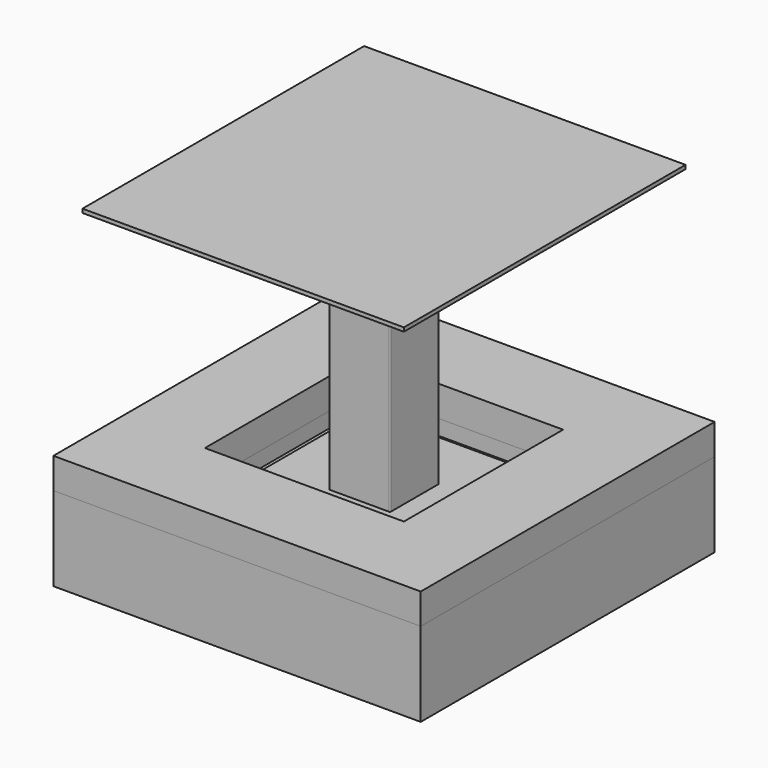
from build123d import *

# Parameters (mm, degrees)
F0_W           = 1219.2
F0_H           = 1219.2
F1_DEPTH       = 304.8
F2_DEPTH       = 25.4
F3_W           = 660.4
F3_H           = 660.4
F4_DEPTH       = 152.4
F5_W           = 660.4
F5_H           = 660.4
F6_DEPTH       = 101.6
F7_W           = 1219.2
F7_H           = 1219.2
F7_W_2         = 660.4
F7_H_2         = 660.4
F8_DEPTH       = 101.6
F9_W           = 609.6
F9_H           = 609.6
F10_DEPTH      = 12.7
F12_DEPTH      = 863.6
F13_W          = 1066.8
F13_H          = 1168.4
F14_DEPTH      = 12.7
F15_R          = 6.35
F16_DEPTH      = 76.2
F17_R          = 6.35
F18_DEPTH      = 50.8
F18_DEPTH_BACK = 12.7


with BuildPart() as f1:
    # F0 (on Top) → F1 (new body)
    with BuildSketch(Plane.XY):
        Rectangle(F0_W, F0_H)
    extrude(amount=-F1_DEPTH)

    # F2 (cut): a face of the model
    f2_faces = [f1.faces().sort_by_distance(p)[0] for p in [
        (0, 0, 0),
    ]]
    extrude(f2_faces, amount=-F2_DEPTH, mode=Mode.SUBTRACT)

    # F3 (on face) → F4 (cut)
    with BuildSketch(Plane.XY.offset(-25.4)):
        Rectangle(F3_W, F3_H)
    extrude(amount=-F4_DEPTH, mode=Mode.SUBTRACT)


with BuildPart() as f6:
    # F5 (on face) → F6 (new body)
    with BuildSketch(Plane.XY.offset(-177.8)):
        Rectangle(F5_W, F5_H)
    extrude(amount=F6_DEPTH)


with BuildPart() as f8:
    # F7 (on face) → F8 (new body)
    with BuildSketch(Plane.XY.offset(-25.4)):
        Rectangle(F7_W, F7_H)
        Rectangle(F7_W_2, F7_H_2, mode=Mode.SUBTRACT)
    extrude(amount=F8_DEPTH)


with BuildPart() as f10:
    # F9 (on face) → F10 (new body)
    with BuildSketch(Plane.XY.offset(-76.2)):
        Rectangle(F9_W, F9_H)
    extrude(amount=F10_DEPTH)

    # F11 (on face) → F12 (join)
    with BuildSketch(Plane.XY.offset(-63.5)):
        with BuildLine():
            ThreePointArc((-101.6, -98.425), (-100.6700640303, -100.6700640303), (-98.425, -101.6))
            Line((-98.425, -101.6), (98.425, -101.6))
            ThreePointArc((98.425, -101.6), (100.6700640303, -100.6700640303), (101.6, -98.425))
            Line((101.6, -98.425), (101.6, 98.425))
            ThreePointArc((101.6, 98.425), (100.6700640303, 100.6700640303), (98.425, 101.6))
            Line((98.425, 101.6), (-98.425, 101.6))
            ThreePointArc((-98.425, 101.6), (-100.6700640303, 100.6700640303), (-101.6, 98.425))
            Line((-101.6, 98.425), (-101.6, -98.425))
        make_face()
        with BuildLine():
            ThreePointArc((-95.25, 92.075), (-94.3200640303, 94.3200640303), (-92.075, 95.25))
            Line((-92.075, 95.25), (92.075, 95.25))
            ThreePointArc((92.075, 95.25), (94.3200640303, 94.3200640303), (95.25, 92.075))
            Line((95.25, 92.075), (95.25, -92.075))
            ThreePointArc((95.25, -92.075), (94.3200640303, -94.3200640303), (92.075, -95.25))
            Line((92.075, -95.25), (-92.075, -95.25))
            ThreePointArc((-92.075, -95.25), (-94.3200640303, -94.3200640303), (-95.25, -92.075))
            Line((-95.25, -92.075), (-95.25, 92.075))
        make_face(mode=Mode.SUBTRACT)
    extrude(amount=F12_DEPTH)

    # F13 (on face) → F14 (join)
    with BuildSketch(Plane.XY.offset(800.1)):
        Rectangle(F13_W, F13_H)
    extrude(amount=F14_DEPTH)

    # F15 (on face) → F16 (cut)
    with BuildSketch(Plane.XY.offset(-63.5)):
        with Locations((-264.3490433693, 264.3490433693)):
            Circle(F15_R)
        with Locations((252.229899168, 264.3490433693)):
            Circle(F15_R)
        with Locations((252.229899168, -259.8043680191)):
            Circle(F15_R)
        with Locations((-264.3490433693, -259.8043680191)):
            Circle(F15_R)
    extrude(amount=-F16_DEPTH, mode=Mode.SUBTRACT)


with BuildPart() as f18:
    # F17 (on face) → F18 (new body, two sides)
    with BuildSketch(Plane.XY.offset(-63.5)) as f18_sk:
        with Locations((-264.3490433693, 264.3490433693)):
            Circle(F17_R)
    extrude(amount=-F18_DEPTH)
    extrude(f18_sk.sketch, amount=F18_DEPTH_BACK)


with BuildPart() as f18b:
    # F17 (on face) → F18, piece 2 (new body, two sides)
    with BuildSketch(Plane.XY.offset(-63.5)) as f18_2_sk:
        with Locations((252.229899168, 264.3490433693)):
            Circle(F17_R)
    extrude(amount=-F18_DEPTH)
    extrude(f18_2_sk.sketch, amount=F18_DEPTH_BACK)


with BuildPart() as f18c:
    # F17 (on face) → F18, piece 3 (new body, two sides)
    with BuildSketch(Plane.XY.offset(-63.5)) as f18_3_sk:
        with Locations((252.229899168, -259.8043680191)):
            Circle(F17_R)
    extrude(amount=-F18_DEPTH)
    extrude(f18_3_sk.sketch, amount=F18_DEPTH_BACK)


with BuildPart() as f18d:
    # F17 (on face) → F18, piece 4 (new body, two sides)
    with BuildSketch(Plane.XY.offset(-63.5)) as f18_4_sk:
        with Locations((-264.3490433693, -259.8043680191)):
            Circle(F17_R)
    extrude(amount=-F18_DEPTH)
    extrude(f18_4_sk.sketch, amount=F18_DEPTH_BACK)


solid = Compound([f1.part, f6.part, f8.part, f10.part, f18.part, f18b.part, f18c.part, f18d.part])
